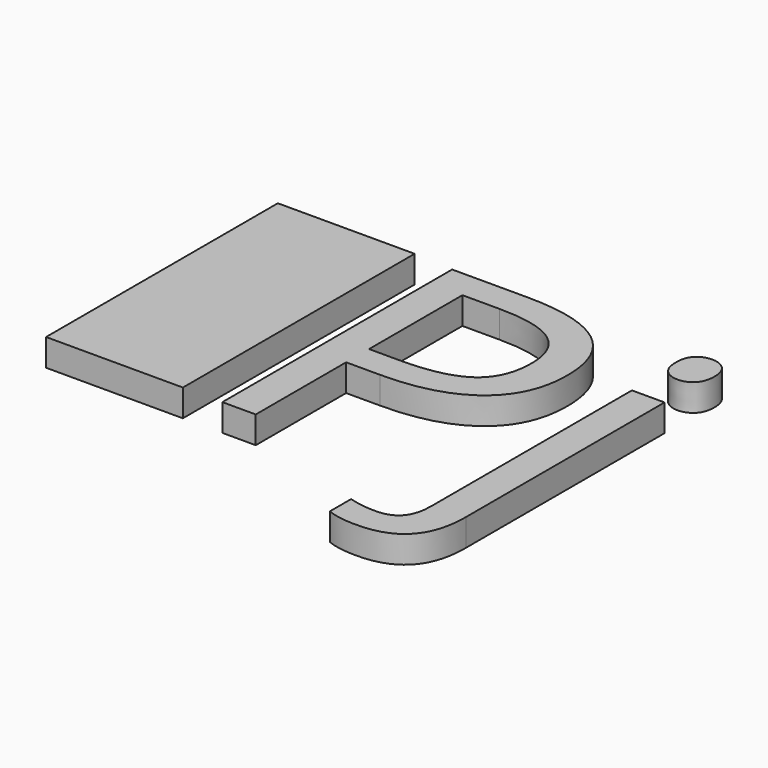
from build123d import *

# Parameters (mm, degrees)
F0_W         = 10.0988904014
F0_H         = 21.3848152961
F0_TEXT_SIZE = 29.7011323557
F1_DEPTH     = 2


# Not quite as in the source:
# - Text() gives the source's letters only with a copy of the font that has no kerning and outlines rounded to 1/6400 em; it was checked with that copy


with BuildPart() as f1:
    # F0 (on Top) → F1 (new body)
    with BuildSketch(Plane.XY):
        with Locations((-5.0494452007, 10.692407648)):
            Rectangle(F0_W, F0_H)
        with Locations((0, 0)):
            Text('Pj', F0_TEXT_SIZE, font='Open Sans', text_align=(TextAlign.LEFT, TextAlign.BOTTOM))
    extrude(amount=F1_DEPTH)


solid = f1.part
